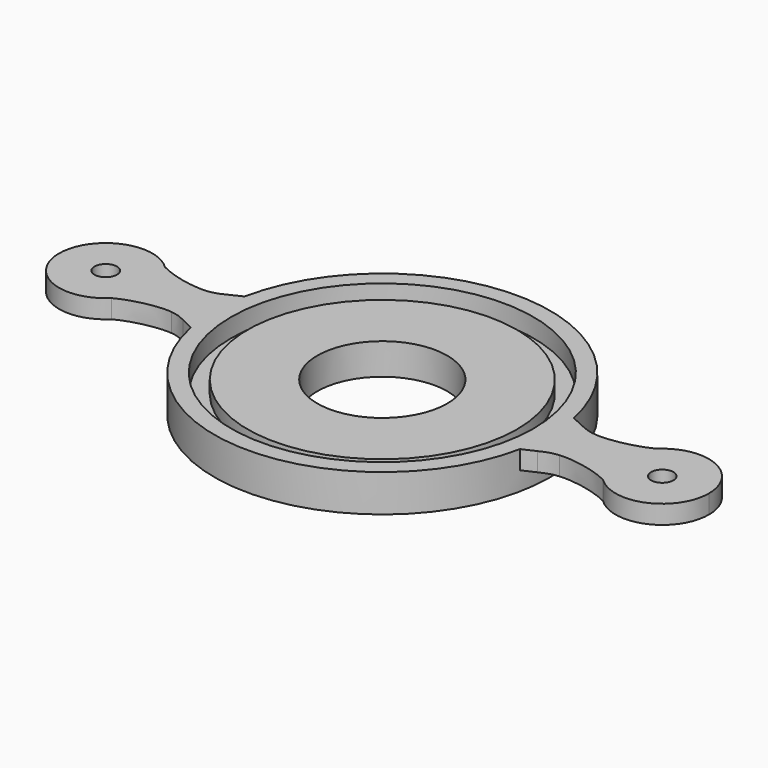
from build123d import *

# Parameters (mm, degrees)
F0_R        = 45
F0_R_2      = 40.5
F1_DEPTH    = 10
F0_R_3      = 36.1
F2_DEPTH    = 5
F0_R_4      = 31
F3_DEPTH    = 8.4
F0_R_5      = 17.4
F4_DEPTH    = 8.4
F5_R        = 3
F1_FACE_R   = 45
F1_FACE_R_2 = 40.5
F6_DEPTH    = 5


with BuildPart() as f1:
    # F0 (on Top) → F1 (new body)
    with BuildSketch(Plane.XY):
        Circle(F0_R)
        Circle(F0_R_2, mode=Mode.SUBTRACT)
    extrude(amount=F1_DEPTH)

    # F0 (on Top) → F2 (join)
    with BuildSketch(Plane.XY):
        Circle(F0_R_2)
        Circle(F0_R_3, mode=Mode.SUBTRACT)
    extrude(amount=F2_DEPTH)

    # F0 (on Top) → F3 (join)
    with BuildSketch(Plane.XY):
        Circle(F0_R_3)
        Circle(F0_R_4, mode=Mode.SUBTRACT)
    extrude(amount=F3_DEPTH)

    # F0 (on Top) → F4 (join)
    with BuildSketch(Plane.XY):
        Circle(F0_R_4)
        Circle(F0_R_5, mode=Mode.SUBTRACT)
    extrude(amount=F4_DEPTH)

    # F5 (on face) + F1_face (on face) → F6 (join)
    with BuildSketch(Plane.XY.offset(10)):
        with BuildLine():
            ThreePointArc((66.3253242136, -9), (79.8896090165, -11.5039872942), (87.5, 0))
            ThreePointArc((87.5, 0), (79.8896090165, 11.5039872942), (66.3253242136, 9))
            Line((66.3253242136, 9), (66.3253242136, 0))
            Line((66.3253242136, 0), (66.3253242136, -9))
        make_face()
        with BuildLine():
            ThreePointArc((78, 0), (75, -3), (72, 0))
            ThreePointArc((72, 0), (75, 3), (78, 0))
        make_face(mode=Mode.SUBTRACT)
        with BuildLine():
            ThreePointArc((62.5527321378, -1.1469624085), (63.7327165773, -5.4127926501), (66.3253242136, -9))
            Line((66.3253242136, -9), (66.3253242136, 0))
            Line((66.3253242136, 0), (62.5527321378, 0))
            Line((62.5527321378, 0), (62.5527321378, -1.1469624085))
        make_face()
        with BuildLine():
            Line((66.3253242136, 0), (66.3253242136, 9))
            ThreePointArc((66.3253242136, 9), (63.7327165773, 5.4127926501), (62.5527321378, 1.1469624085))
            Line((62.5527321378, 1.1469624085), (62.5527321378, 0))
            Line((62.5527321378, 0), (66.3253242136, 0))
        make_face()
        with BuildLine():
            ThreePointArc((62.5527321378, 1.1469624085), (63.7327165773, 5.4127926501), (66.3253242136, 9))
            add(Edge.make_bspline(
                [(66.3253242136, 9), (62.5527321378, 7.0294414229), (56.1633100825, 5.6459116487), (52.2136635361, 6)],
                knots=[0, 0, 0, 0, 0.5634667873, 0.5634667873, 0.5634667873, 0.5634667873], degree=3))
            Line((52.2136635361, 6), (52.2136635361, 0))
            Line((52.2136635361, 0), (62.5, 0))
            ThreePointArc((62.5, 0), (62.5131899935, 0.5740869806), (62.5527321378, 1.1469624085))
        make_face()
        with BuildLine():
            add(Edge.make_bspline(
                [(52.2136635361, -6), (50.3742603721, -6.1649036758), (49.0640175166, -6.7066774941), (47.5582238129, -7.4185810788)],
                knots=[0.5634667873, 0.5634667873, 0.5634667873, 0.5634667873, 0.8258807981, 0.8258807981, 0.8258807981, 0.8258807981], degree=3))
            Line((52.2136635361, -6), (52.2136635361, 0))
            Line((52.2136635361, 0), (47.5582238129, 0))
            Line((47.5582238129, 0), (47.5582238129, -7.4185810788))
        make_face()
        with BuildLine():
            Line((62.5527321378, 0), (62.5527321378, 1.1469624085))
            ThreePointArc((62.5527321378, 1.1469624085), (62.5131899935, 0.5740869806), (62.5, 0))
            Line((62.5, 0), (62.5527321378, 0))
        make_face()
        with BuildLine():
            ThreePointArc((62.5, 0), (62.5131899935, -0.5740869806), (62.5527321378, -1.1469624085))
            Line((62.5527321378, -1.1469624085), (62.5527321378, 0))
            Line((62.5527321378, 0), (62.5, 0))
        make_face()
        with BuildLine():
            add(Edge.make_bspline(
                [(66.3253242136, -9), (62.5527321378, -7.0294414229), (56.1633100825, -5.6459116487), (52.2136635361, -6)],
                knots=[0, 0, 0, 0, 0.5634667873, 0.5634667873, 0.5634667873, 0.5634667873], degree=3))
            ThreePointArc((66.3253242136, -9), (63.7327165773, -5.4127926501), (62.5527321378, -1.1469624085))
            ThreePointArc((62.5527321378, -1.1469624085), (62.5131899935, -0.5740869806), (62.5, 0))
            Line((62.5, 0), (52.2136635361, 0))
            Line((52.2136635361, 0), (52.2136635361, -6))
        make_face()
        with BuildLine():
            Line((52.2136635361, 0), (52.2136635361, 6))
            add(Edge.make_bspline(
                [(52.2136635361, 6), (50.3742603721, 6.1649036758), (49.0640175166, 6.7066774941), (47.5582238129, 7.4185810788)],
                knots=[0.5634667873, 0.5634667873, 0.5634667873, 0.5634667873, 0.8258807981, 0.8258807981, 0.8258807981, 0.8258807981], degree=3))
            Line((47.5582238129, 7.4185810788), (47.5582238129, 0))
            Line((47.5582238129, 0), (52.2136635361, 0))
        make_face()
        with BuildLine():
            add(Edge.make_bspline(
                [(47.5582238129, -7.4185810788), (46.5590866207, -7.8909494696), (45.4738542162, -8.4382209279), (44.0908153701, -9)],
                knots=[0.8258807981, 0.8258807981, 0.8258807981, 0.8258807981, 1, 1, 1, 1], degree=3))
            Line((47.5582238129, -7.4185810788), (47.5582238129, 0))
            Line((47.5582238129, 0), (45, 0))
            ThreePointArc((45, 0), (44.7721268852, -4.5229032902), (44.0908153701, -9))
        make_face()
        with BuildLine():
            Line((47.5582238129, 0), (47.5582238129, 7.4185810788))
            add(Edge.make_bspline(
                [(47.5582238129, 7.4185810788), (46.5590866207, 7.8909494696), (45.4738542162, 8.4382209279), (44.0908153701, 9)],
                knots=[0.8258807981, 0.8258807981, 0.8258807981, 0.8258807981, 1, 1, 1, 1], degree=3))
            ThreePointArc((44.0908153701, 9), (44.7721268852, 4.5229032902), (45, 0))
            Line((45, 0), (47.5582238129, 0))
        make_face()
        with BuildLine():
            ThreePointArc((-44.0908153701, -9), (0, -45), (44.0908153701, -9))
            Line((44.0908153701, -9), (44.0908153701, 0))
            Line((44.0908153701, 0), (40.5, 0))
            ThreePointArc((40.5, 0), (0, -40.5), (-40.5, 0))
            Line((-40.5, 0), (-44.0908153701, 0))
            Line((-44.0908153701, 0), (-44.0908153701, -9))
        make_face()
        with BuildLine():
            Line((-51.7064335188, 0), (-51.7064335188, 6))
            add(Edge.make_bspline(
                [(-65.4197458811, 9.0034745469), (-61.6860010238, 6.9482695309), (-55.4334302889, 5.6320399313), (-51.7064335188, 6)],
                knots=[0, 0, 0, 0, 0.567027295, 0.567027295, 0.567027295, 0.567027295], degree=3))
            ThreePointArc((-65.4197458811, 9.0034745469), (-62.911579364, 5.5923771619), (-61.6860010238, 1.5396691315))
            ThreePointArc((-61.6860010238, 1.5396691315), (-61.6146344775, 0.7713043082), (-61.5908153701, 0))
            Line((-61.5908153701, 0), (-51.7064335188, 0))
        make_face()
        with BuildLine():
            ThreePointArc((-45, 0), (-44.7721268852, -4.5229032902), (-44.0908153701, -9))
            Line((-44.0908153701, -9), (-44.0908153701, 0))
            Line((-44.0908153701, 0), (-45, 0))
        make_face()
        with BuildLine():
            add(Edge.make_bspline(
                [(-65.4125331798, -8.996522563), (-61.6860010238, -6.9482695309), (-55.4331204309, -5.6323249689), (-51.7064335188, -6)],
                knots=[0, 0, 0, 0, 0.566952665, 0.566952665, 0.566952665, 0.566952665], degree=3))
            Line((-51.7064335188, -6), (-51.7064335188, 0))
            Line((-51.7064335188, 0), (-61.5908153701, 0))
            ThreePointArc((-61.5908153701, 0), (-61.6146344775, -0.7713043082), (-61.6860010238, -1.5396691315))
            ThreePointArc((-61.6860010238, -1.5396691315), (-62.9093393644, -5.5878971298), (-65.4125331798, -8.996522563))
        make_face()
        with BuildLine():
            add(Edge.make_bspline(
                [(-51.7064335188, -6), (-50.0263203675, -6.1657600088), (-48.8596569, -6.6737162451), (-47.4872474781, -7.3615768954)],
                knots=[0.566952665, 0.566952665, 0.566952665, 0.566952665, 0.8225535918, 0.8225535918, 0.8225535918, 0.8225535918], degree=3))
            Line((-47.4872474781, -7.3615768954), (-47.4872474781, 0))
            Line((-47.4872474781, 0), (-51.7064335188, 0))
            Line((-51.7064335188, 0), (-51.7064335188, -6))
        make_face()
        with BuildLine():
            ThreePointArc((-61.6860010238, 1.5396691315), (-62.911579364, 5.5923771619), (-65.4197458811, 9.0034745469))
            Line((-65.4197458811, 9.0034745469), (-65.4197458811, 0.0034745469))
            Line((-65.4197458811, 0.0034745469), (-65.4197430965, 0))
            Line((-65.4197430965, 0), (-61.6860010238, 0))
            Line((-61.6860010238, 0), (-61.6860010238, 1.5396691315))
        make_face()
        with BuildLine():
            Line((-65.4197430965, 0), (-65.4125331798, -8.996522563))
            ThreePointArc((-65.4125331798, -8.996522563), (-62.9093393644, -5.5878971298), (-61.6860010238, -1.5396691315))
            Line((-61.6860010238, -1.5396691315), (-61.6860010238, 0))
            Line((-61.6860010238, 0), (-65.4197430965, 0))
        make_face()
        with BuildLine():
            add(Edge.make_bspline(
                [(-47.4872474781, -7.3615768954), (-46.5344765882, -7.8391119468), (-45.482544702, -8.4033534464), (-44.0908153701, -9)],
                knots=[0.8225535918, 0.8225535918, 0.8225535918, 0.8225535918, 1, 1, 1, 1], degree=3))
            ThreePointArc((-44.0908153701, -9), (-44.7721268852, -4.5229032902), (-45, 0))
            Line((-45, 0), (-47.4872474781, 0))
            Line((-47.4872474781, 0), (-47.4872474781, -7.3615768954))
        make_face()
        with BuildLine():
            ThreePointArc((-45, 0), (-44.7721268852, 4.5229032902), (-44.0908153701, 9))
            add(Edge.make_bspline(
                [(-47.4872474781, 7.3617098784), (-46.5344445734, 7.8392079283), (-45.4824537219, 8.4033924504), (-44.0908153701, 9)],
                knots=[0.8225957704, 0.8225957704, 0.8225957704, 0.8225957704, 1, 1, 1, 1], degree=3))
            Line((-47.4872474781, 7.3617098784), (-47.4872474781, 0))
            Line((-47.4872474781, 0), (-45, 0))
        make_face()
        with BuildLine():
            Line((-44.0908153701, 0), (-44.0908153701, 9))
            ThreePointArc((-44.0908153701, 9), (-44.7721268852, 4.5229032902), (-45, 0))
            Line((-45, 0), (-44.0908153701, 0))
        make_face()
        with BuildLine():
            ThreePointArc((-61.6860010238, -1.5396691315), (-61.6146344775, -0.7713043082), (-61.5908153701, 0))
            Line((-61.5908153701, 0), (-61.6860010238, 0))
            Line((-61.6860010238, 0), (-61.6860010238, -1.5396691315))
        make_face()
        with BuildLine():
            ThreePointArc((-61.5908153701, 0), (-61.6146344775, 0.7713043082), (-61.6860010238, 1.5396691315))
            Line((-61.6860010238, 1.5396691315), (-61.6860010238, 0))
            Line((-61.6860010238, 0), (-61.5908153701, 0))
        make_face()
        with BuildLine():
            Line((-47.4872474781, 0), (-47.4872474781, 7.3617098784))
            add(Edge.make_bspline(
                [(-51.7064335188, 6), (-50.0266151205, 6.1658456208), (-48.8598550323, 6.6738263432), (-47.4872474781, 7.3617098784)],
                knots=[0.567027295, 0.567027295, 0.567027295, 0.567027295, 0.8225957704, 0.8225957704, 0.8225957704, 0.8225957704], degree=3))
            Line((-51.7064335188, 6), (-51.7064335188, 0))
            Line((-51.7064335188, 0), (-47.4872474781, 0))
        make_face()
        with BuildLine():
            Line((-65.4197458811, 0.0034745469), (-65.4197458811, 9.0034745469))
            ThreePointArc((-65.4197458811, 9.0034745469), (-86.5908143666, -0.0050088207), (-65.4125331798, -8.996522563))
            Line((-65.4125331798, -8.996522563), (-65.4197430965, 0))
            Line((-65.4197430965, 0), (-65.4197458811, 0.0034745469))
        make_face()
        with Locations((-74.0908153701, 0)):
            Circle(F5_R, mode=Mode.SUBTRACT)
    with BuildSketch(Plane.XY.offset(10)):
        Circle(F1_FACE_R)
        Circle(F1_FACE_R_2, mode=Mode.SUBTRACT)
    extrude(amount=-F6_DEPTH)


solid = f1.part
